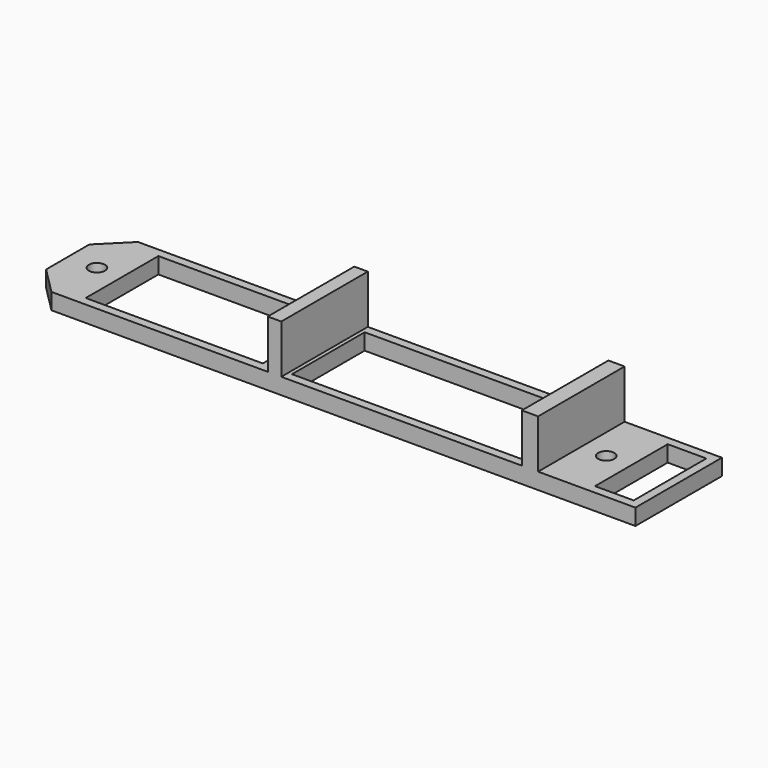
from build123d import *

# Parameters (mm, degrees)
F0_W      = 113
F0_H      = 20
F1_DEPTH  = 3
F2_W      = 2.5
F2_H      = 20
F2_W_2    = 3
F3_DEPTH  = 12
F4_R      = 1.5
F5_DEPTH  = 3
F6_R      = 3.05
F6_R_2    = 1.5
F7_DEPTH  = 1
F8_W      = 32.75
F8_H      = 16.8
F8_W_2    = 43.6
F8_W_3    = 7.15
F9_DEPTH  = 3
F10_SIZE  = 5
F11_ANGLE = 180


# Not quite as in the source:
# - a feature of the source that left no trace in its solid (it failed there, or was rolled back) is left out


with BuildPart() as f1:
    # F0 (on Top) → F1 (new body)
    with BuildSketch(Plane.XY):
        Rectangle(F0_W, F0_H)
    extrude(amount=F1_DEPTH)

    # F2 (on face) → F3 (join)
    with BuildSketch(Plane.XY.offset(3)):
        with Locations((-10.25, 0)):
            Rectangle(F2_W, F2_H)
        with Locations((37, 0)):
            Rectangle(F2_W_2, F2_H)
    extrude(amount=-F3_DEPTH)

    # F4 (on face) → F5 (cut, through all)
    with BuildSketch(Plane.XY.offset(3)):
        with Locations((-51.1, 0)):
            Circle(F4_R)
        with Locations((43.1, 0)):
            Circle(F4_R)
    extrude(amount=-F5_DEPTH, mode=Mode.SUBTRACT)

    # F6 (on face) → F7 (cut)
    with BuildSketch(Plane.XY.offset(3)):
        with Locations((-51.1, 0)):
            Circle(F6_R)
        with Locations((-51.1, 0)):
            Circle(F6_R_2, mode=Mode.SUBTRACT)
        with Locations((43.1, 0)):
            Circle(F6_R)
        with Locations((43.1, 0)):
            Circle(F6_R_2, mode=Mode.SUBTRACT)
    extrude(amount=-F7_DEPTH, mode=Mode.SUBTRACT)

    # F8 (on face) → F9 (cut, through all)
    with BuildSketch(Plane.XY.offset(3)):
        with Locations((-30.075, 0)):
            Rectangle(F8_W, F8_H)
        with Locations((13.5, 0)):
            Rectangle(F8_W_2, F8_H)
        with Locations((51.325, 0)):
            Rectangle(F8_W_3, F8_H)
    extrude(amount=-F9_DEPTH, mode=Mode.SUBTRACT)

    # F10
    f10_edges = [f1.edges().sort_by_distance(p)[0] for p in [
        (-56.5, 10, 1.5),
        (-56.5, -10, 1.5),
    ]]
    chamfer(f10_edges, length=F10_SIZE)


with BuildPart() as f1_1:
    # F11: moved
    add(f1.part.rotate(Axis((2.5, -10, 3), (-1, 0, 0)), F11_ANGLE))


solid = f1_1.part
